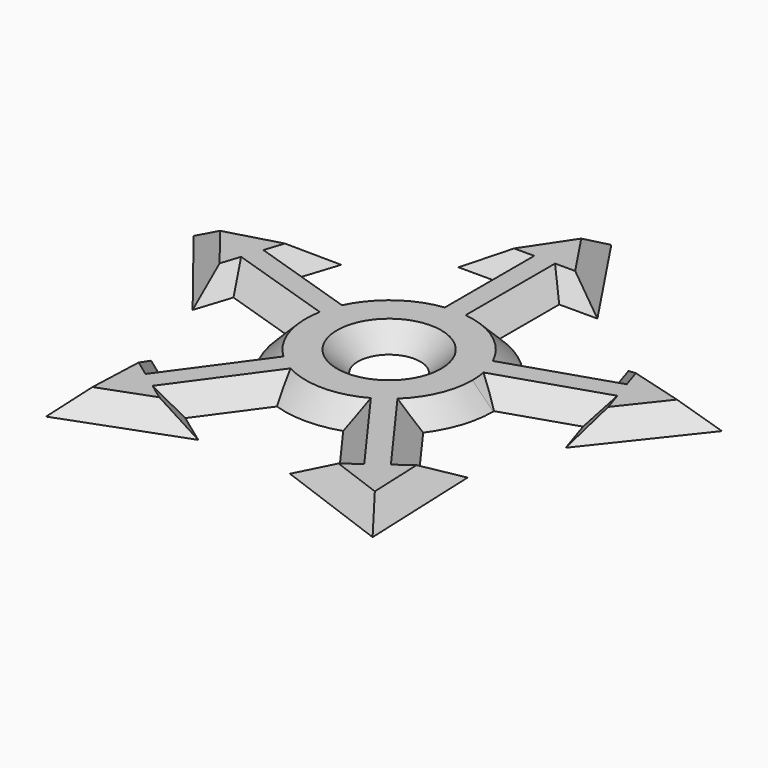
from build123d import *

# Parameters (mm, degrees)
F0_R     = 4.5
F1_DEPTH = 3
F2_SIZE2 = 2.99999
F2_SIZE  = 2.99999


# Not quite as in the source:
# - a fillet or chamfer is up to 0.001 mm smaller than in the source, because OpenCascade refuses the exact size


with BuildPart() as f1:
    # F0 (on Top) → F1 (new body)
    with BuildSketch(Plane.XY):
        with BuildLine():
            ThreePointArc((12.0512473873, -8.9312617479), (14.2437479409, -4.7027273571), (15, 0))
            ThreePointArc((15, 0), (14.9998319689, 0.07099932), (14.9993278795, 0.1419970492))
            Line((14.9993278795, 0.1419970492), (9.794719653, -1.5490826747))
            Line((9.794719653, -1.5490826747), (7.0135667036, 7.0104259719))
            Line((7.0135667036, 7.0104259719), (12.2181749302, 8.7015056959))
            ThreePointArc((12.2181749302, 8.7015056959), (8.8167787844, 12.1352549156), (4.5, 14.3090880213))
            Line((4.5, 14.3090880213), (4.5, 8.8366390791))
            Line((4.5, 8.8366390791), (-4.5, 8.8366390791))
            Line((-4.5, 8.8366390791), (-4.5, 14.3090880213))
            ThreePointArc((-4.5, 14.3090880213), (-8.8167787844, 12.1352549156), (-12.2181749302, 8.7015056959))
            Line((-12.2181749302, 8.7015056959), (-7.0135667036, 7.0104259719))
            Line((-7.0135667036, 7.0104259719), (-9.794719653, -1.5490826747))
            Line((-9.794719653, -1.5490826747), (-14.9993278795, 0.1419970492))
            ThreePointArc((-14.9993278795, 0.1419970492), (-14.2658477444, -4.6352549156), (-12.0512473873, -8.9312617479))
            Line((-12.0512473873, -8.9312617479), (-8.8346226052, -4.5039575528))
            Line((-8.8346226052, -4.5039575528), (-1.5534696558, -9.7940248235))
            Line((-1.5534696558, -9.7940248235), (-4.770094438, -14.2213290185))
            ThreePointArc((-4.770094438, -14.2213290185), (0, -15), (4.770094438, -14.2213290185))
            Line((4.770094438, -14.2213290185), (1.5534696558, -9.7940248235))
            Line((1.5534696558, -9.7940248235), (8.8346226052, -4.5039575528))
            Line((8.8346226052, -4.5039575528), (12.0512473873, -8.9312617479))
        make_face()
        Circle(F0_R, mode=Mode.SUBTRACT)
        with BuildLine():
            Line((9.794719653, -1.5490826747), (14.9993278795, 0.1419970492))
            ThreePointArc((14.9993278795, 0.1419970492), (14.2658477444, 4.6352549156), (12.2181749302, 8.7015056959))
            Line((12.2181749302, 8.7015056959), (7.0135667036, 7.0104259719))
            Line((7.0135667036, 7.0104259719), (9.794719653, -1.5490826747))
        make_face()
        with BuildLine():
            ThreePointArc((12.2181749302, 8.7015056959), (14.2658477444, 4.6352549156), (14.9993278795, 0.1419970492))
            Line((14.9993278795, 0.1419970492), (25.1669893821, 3.445670536))
            Line((25.1669893821, 3.445670536), (22.3858364327, 12.0051791827))
            Line((22.3858364327, 12.0051791827), (12.2181749302, 8.7015056959))
        make_face()
        with BuildLine():
            Line((18.335207782, -17.5803912241), (12.0512473873, -8.9312617479))
            ThreePointArc((12.0512473873, -8.9312617479), (8.8167787844, -12.1352549156), (4.770094438, -14.2213290185))
            Line((4.770094438, -14.2213290185), (11.0540548326, -22.8704584947))
            Line((11.0540548326, -22.8704584947), (18.335207782, -17.5803912241))
        make_face()
        with BuildLine():
            ThreePointArc((4.770094438, -14.2213290185), (8.8167787844, -12.1352549156), (12.0512473873, -8.9312617479))
            Line((12.0512473873, -8.9312617479), (8.8346226052, -4.5039575528))
            Line((8.8346226052, -4.5039575528), (1.5534696558, -9.7940248235))
            Line((1.5534696558, -9.7940248235), (4.770094438, -14.2213290185))
        make_face()
        Polygon((22.3858364327, 12.0051791827), (25.1669893821, 3.445670536), (26.8665828511, -1.7851403036), (38.0422606518, 12.360679775), (20.6862429636, 17.2359900223), align=None)
        Polygon((22.7848012511, -14.3475723364), (18.335207782, -17.5803912241), (11.0540548326, -22.8704584947), (6.6044613636, -26.1032773823), (23.5114100917, -32.360679775), align=None)
        with BuildLine():
            Line((4.5, 8.8366390791), (4.5, 14.3090880213))
            ThreePointArc((4.5, 14.3090880213), (0, 15), (-4.5, 14.3090880213))
            Line((-4.5, 14.3090880213), (-4.5, 8.8366390791))
            Line((-4.5, 8.8366390791), (4.5, 8.8366390791))
        make_face()
        with BuildLine():
            ThreePointArc((-4.5, 14.3090880213), (0, 15), (4.5, 14.3090880213))
            Line((4.5, 14.3090880213), (4.5, 25))
            Line((4.5, 25), (-4.5, 25))
            Line((-4.5, 25), (-4.5, 14.3090880213))
        make_face()
        with BuildLine():
            Line((-11.0540548326, -22.8704584947), (-4.770094438, -14.2213290185))
            ThreePointArc((-4.770094438, -14.2213290185), (-8.8167787844, -12.1352549156), (-12.0512473873, -8.9312617479))
            Line((-12.0512473873, -8.9312617479), (-18.335207782, -17.5803912241))
            Line((-18.335207782, -17.5803912241), (-11.0540548326, -22.8704584947))
        make_face()
        with BuildLine():
            ThreePointArc((-12.0512473873, -8.9312617479), (-8.8167787844, -12.1352549156), (-4.770094438, -14.2213290185))
            Line((-4.770094438, -14.2213290185), (-1.5534696558, -9.7940248235))
            Line((-1.5534696558, -9.7940248235), (-8.8346226052, -4.5039575528))
            Line((-8.8346226052, -4.5039575528), (-12.0512473873, -8.9312617479))
        make_face()
        Polygon((-4.5, 25), (4.5, 25), (10, 25), (0, 40), (-10, 25), align=None)
        Polygon((-6.6044613636, -26.1032773823), (-11.0540548326, -22.8704584947), (-18.335207782, -17.5803912241), (-22.7848012511, -14.3475723364), (-23.5114100917, -32.360679775), align=None)
        with BuildLine():
            Line((-7.0135667036, 7.0104259719), (-12.2181749302, 8.7015056959))
            ThreePointArc((-12.2181749302, 8.7015056959), (-14.2658477444, 4.6352549156), (-14.9993278795, 0.1419970492))
            Line((-14.9993278795, 0.1419970492), (-9.794719653, -1.5490826747))
            Line((-9.794719653, -1.5490826747), (-7.0135667036, 7.0104259719))
        make_face()
        with BuildLine():
            ThreePointArc((-14.9993278795, 0.1419970492), (-14.2658477444, 4.6352549156), (-12.2181749302, 8.7015056959))
            Line((-12.2181749302, 8.7015056959), (-22.3858364327, 12.0051791827))
            Line((-22.3858364327, 12.0051791827), (-25.1669893821, 3.445670536))
            Line((-25.1669893821, 3.445670536), (-14.9993278795, 0.1419970492))
        make_face()
        Polygon((-25.1669893821, 3.445670536), (-22.3858364327, 12.0051791827), (-20.6862429636, 17.2359900223), (-38.0422606518, 12.360679775), (-26.8665828511, -1.7851403036), align=None)
    extrude(amount=F1_DEPTH)

    # F2 (size 3 and 3 in the source; OpenCascade refuses exactly that, so slightly less here)
    f2_edges = [f1.edges().sort_by_distance(p)[0] for p in [
        (-15.193228, -13.255826, 3),
        (-20.560005, -15.963982, 3),
        (-23.148106, -23.354126, 3),
        (-15.057936, -29.231979, 3),
        (-8.829258, -24.486868, 3),
        (-7.912075, -18.545894, 3),
        (0, -15, 3),
        (7.912075, -18.545894, 3),
        (8.829258, -24.486868, 3),
        (15.057936, -29.231979, 3),
        (23.148106, -23.354126, 3),
        (20.560005, -15.963982, 3),
        (15.193228, -13.255826, 3),
        (14.265848, -4.635255, 3),
        (20.083159, 1.793834, 3),
        (26.016786, 0.830265, 3),
        (32.454422, 5.28777, 3),
        (29.364252, 14.798335, 3),
        (21.53604, 14.620585, 3),
        (17.302006, 10.353342, 3),
        (8.816779, 12.135255, 3),
        (4.5, 19.654544, 3),
        (7.25, 25, 3),
        (5, 32.5, 3),
        (-5, 32.5, 3),
        (-7.25, 25, 3),
        (-4.5, 19.654544, 3),
        (-8.816779, 12.135255, 3),
        (-17.302006, 10.353342, 3),
        (-21.53604, 14.620585, 3),
        (-29.364252, 14.798335, 3),
        (-32.454422, 5.28777, 3),
        (-26.016786, 0.830265, 3),
        (-20.083159, 1.793834, 3),
        (-14.265848, -4.635255, 3),
        (-4.5, 0, 3),
    ]]
    chamfer(f2_edges, length=F2_SIZE, length2=F2_SIZE2)


solid = f1.part
